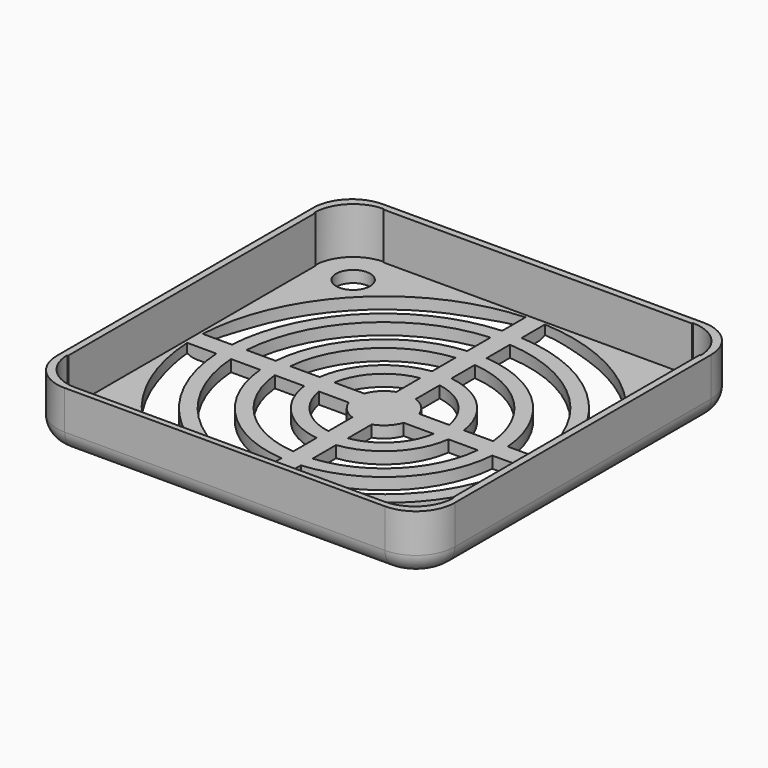
from build123d import *

# Parameters (mm, degrees)
F0_R         = 1.75
F1_DEPTH     = 1.2
F2_DEPTH     = 6
F4_DEPTH     = 10
F5_T1_DEPTH  = 33
F5_T3_DEPTH  = 33
F5_T6_ANGLE  = 90
F5_T8_ANGLE  = 90
F5_T10_ANGLE = 90
F5_T12_ANGLE = 90
F6_DEPTH     = 0.1
F7_DEPTH     = 0.1
F8_DEPTH     = 0.1


# Not quite as in the source:
# - a fillet or chamfer that OpenCascade refuses, or shapes differently, is made with other operations: its cross-section is extruded or revolved along the edge and cut away or added


with BuildPart() as f1:
    # F0 (on Top) → F1 (new body)
    with BuildSketch(Plane.XY):
        with BuildLine():
            Line((-15.9, -19.9), (15.9, -19.9))
            ThreePointArc((15.9, -19.9), (18.7284271247, -18.7284271247), (19.9, -15.9))
            Line((19.9, -15.9), (19.9, 15.9))
            ThreePointArc((19.9, 15.9), (18.7284271247, 18.7284271247), (15.9, 19.9))
            Line((15.9, 19.9), (-15.9, 19.9))
            ThreePointArc((-15.9, 19.9), (-18.7284271247, 18.7284271247), (-19.9, 15.9))
            Line((-19.9, 15.9), (-19.9, -15.9))
            ThreePointArc((-19.9, -15.9), (-18.7284271247, -18.7284271247), (-15.9, -19.9))
        make_face()
        with Locations((-15.9, -15.9)):
            Circle(F0_R, mode=Mode.SUBTRACT)
        with Locations((15.9, -15.9)):
            Circle(F0_R, mode=Mode.SUBTRACT)
        with Locations((-15.9, 15.9)):
            Circle(F0_R, mode=Mode.SUBTRACT)
        with Locations((15.9, 15.9)):
            Circle(F0_R, mode=Mode.SUBTRACT)
    extrude(amount=F1_DEPTH)

    # F0 (on Top) → F2 (join)
    with BuildSketch(Plane.XY):
        with BuildLine():
            Line((-16.5, -20.5), (16.5, -20.5))
            ThreePointArc((16.5, -20.5), (19.3284271247, -19.3284271247), (20.5, -16.5))
            Line((20.5, -16.5), (20.5, 16.5))
            ThreePointArc((20.5, 16.5), (19.3284271247, 19.3284271247), (16.5, 20.5))
            Line((16.5, 20.5), (-16.5, 20.5))
            ThreePointArc((-16.5, 20.5), (-19.3284271247, 19.3284271247), (-20.5, 16.5))
            Line((-20.5, 16.5), (-20.5, -16.5))
            ThreePointArc((-20.5, -16.5), (-19.3284271247, -19.3284271247), (-16.5, -20.5))
        make_face()
        with BuildLine():
            ThreePointArc((19.9, -15.9), (18.7284271247, -18.7284271247), (15.9, -19.9))
            Line((15.9, -19.9), (-15.9, -19.9))
            ThreePointArc((-15.9, -19.9), (-18.7284271247, -18.7284271247), (-19.9, -15.9))
            Line((-19.9, -15.9), (-19.9, 15.9))
            ThreePointArc((-19.9, 15.9), (-18.7284271247, 18.7284271247), (-15.9, 19.9))
            Line((-15.9, 19.9), (15.9, 19.9))
            ThreePointArc((15.9, 19.9), (18.7284271247, 18.7284271247), (19.9, 15.9))
            Line((19.9, 15.9), (19.9, -15.9))
        make_face(mode=Mode.SUBTRACT)
    extrude(amount=F2_DEPTH)

    # F3 (on face) → F4 (cut)
    with BuildSketch(Plane(origin=(0, 0, 0), x_dir=(1, 0, 0), z_dir=(0, 0, -1))):
        with BuildLine():
            ThreePointArc((1, 2.8284271247), (2.1213203436, 2.1213203436), (2.8284271247, 1))
            Line((2.8284271247, 1), (5.9160797831, 1))
            ThreePointArc((5.9160797831, 1), (4.2426406871, 4.2426406871), (1, 5.9160797831))
            Line((1, 5.9160797831), (1, 2.8284271247))
        make_face()
        with BuildLine():
            Line((5.9160797831, -1), (2.8284271247, -1))
            ThreePointArc((2.8284271247, -1), (2.1213203436, -2.1213203436), (1, -2.8284271247))
            Line((1, -2.8284271247), (1, -5.9160797831))
            ThreePointArc((1, -5.9160797831), (4.2426406871, -4.2426406871), (5.9160797831, -1))
        make_face()
        with BuildLine():
            ThreePointArc((-2.8284271247, 1), (-2.1213203436, 2.1213203436), (-1, 2.8284271247))
            Line((-1, 2.8284271247), (-1, 5.9160797831))
            ThreePointArc((-1, 5.9160797831), (-4.2426406871, 4.2426406871), (-5.9160797831, 1))
            Line((-5.9160797831, 1), (-2.8284271247, 1))
        make_face()
        with BuildLine():
            ThreePointArc((1, 7.4330343737), (5.3033008589, 5.3033008589), (7.4330343737, 1))
            Line((7.4330343737, 1), (10.4522724802, 1))
            ThreePointArc((10.4522724802, 1), (7.4246212025, 7.4246212025), (1, 10.4522724802))
            Line((1, 10.4522724802), (1, 7.4330343737))
        make_face()
        with BuildLine():
            Line((-1, -5.9160797831), (-1, -2.8284271247))
            ThreePointArc((-1, -2.8284271247), (-2.1213203436, -2.1213203436), (-2.8284271247, -1))
            Line((-2.8284271247, -1), (-5.9160797831, -1))
            ThreePointArc((-5.9160797831, -1), (-4.2426406871, -4.2426406871), (-1, -5.9160797831))
        make_face()
        with BuildLine():
            Line((10.4522724802, -1), (7.4330343737, -1))
            ThreePointArc((7.4330343737, -1), (5.3033008589, -5.3033008589), (1, -7.4330343737))
            Line((1, -7.4330343737), (1, -10.4522724802))
            ThreePointArc((1, -10.4522724802), (7.4246212025, -7.4246212025), (10.4522724802, -1))
        make_face()
        with BuildLine():
            ThreePointArc((-7.4330343737, 1), (-5.3033008589, 5.3033008589), (-1, 7.4330343737))
            Line((-1, 7.4330343737), (-1, 10.4522724802))
            ThreePointArc((-1, 10.4522724802), (-7.4246212025, 7.4246212025), (-10.4522724802, 1))
            Line((-10.4522724802, 1), (-7.4330343737, 1))
        make_face()
        with BuildLine():
            ThreePointArc((1, 11.9582607431), (8.4852813742, 8.4852813742), (11.9582607431, 1))
            Line((11.9582607431, 1), (14.9666295471, 1))
            ThreePointArc((14.9666295471, 1), (10.6066017178, 10.6066017178), (1, 14.9666295471))
            Line((1, 14.9666295471), (1, 11.9582607431))
        make_face()
        with BuildLine():
            Line((-1, -10.4522724802), (-1, -7.4330343737))
            ThreePointArc((-1, -7.4330343737), (-5.3033008589, -5.3033008589), (-7.4330343737, -1))
            Line((-7.4330343737, -1), (-10.4522724802, -1))
            ThreePointArc((-10.4522724802, -1), (-7.4246212025, -7.4246212025), (-1, -10.4522724802))
        make_face()
        with BuildLine():
            Line((14.9666295471, -1), (11.9582607431, -1))
            ThreePointArc((11.9582607431, -1), (8.4852813742, -8.4852813742), (1, -11.9582607431))
            Line((1, -11.9582607431), (1, -14.9666295471))
            ThreePointArc((1, -14.9666295471), (10.6066017178, -10.6066017178), (14.9666295471, -1))
        make_face()
        with BuildLine():
            ThreePointArc((-11.9582607431, 1), (-8.4852813742, 8.4852813742), (-1, 11.9582607431))
            Line((-1, 11.9582607431), (-1, 14.9666295471))
            ThreePointArc((-1, 14.9666295471), (-10.6066017178, 10.6066017178), (-14.9666295471, 1))
            Line((-14.9666295471, 1), (-11.9582607431, 1))
        make_face()
        with BuildLine():
            ThreePointArc((1, 16.469669092), (11.6672618896, 11.6672618896), (16.469669092, 1))
            Line((16.469669092, 1), (19.4743420942, 1))
            ThreePointArc((19.4743420942, 1), (13.7885822331, 13.7885822331), (1, 19.4743420942))
            Line((1, 19.4743420942), (1, 16.469669092))
        make_face()
        with BuildLine():
            Line((-1, -14.9666295471), (-1, -11.9582607431))
            ThreePointArc((-1, -11.9582607431), (-8.4852813742, -8.4852813742), (-11.9582607431, -1))
            Line((-11.9582607431, -1), (-14.9666295471, -1))
            ThreePointArc((-14.9666295471, -1), (-10.6066017178, -10.6066017178), (-1, -14.9666295471))
        make_face()
        with BuildLine():
            Line((19.4743420942, -1), (16.469669092, -1))
            ThreePointArc((16.469669092, -1), (11.6672618896, -11.6672618896), (1, -16.469669092))
            Line((1, -16.469669092), (1, -19.4743420942))
            ThreePointArc((1, -19.4743420942), (13.7885822331, -13.7885822331), (19.4743420942, -1))
        make_face()
        with BuildLine():
            ThreePointArc((-16.469669092, 1), (-11.6672618896, 11.6672618896), (-1, 16.469669092))
            Line((-1, 16.469669092), (-1, 19.4743420942))
            ThreePointArc((-1, 19.4743420942), (-13.7885822331, 13.7885822331), (-19.4743420942, 1))
            Line((-19.4743420942, 1), (-16.469669092, 1))
        make_face()
        with BuildLine():
            Line((-1, -19.4743420942), (-1, -16.469669092))
            ThreePointArc((-1, -16.469669092), (-11.6672618896, -11.6672618896), (-16.469669092, -1))
            Line((-16.469669092, -1), (-19.4743420942, -1))
            ThreePointArc((-19.4743420942, -1), (-13.7885822331, -13.7885822331), (-1, -19.4743420942))
        make_face()
    extrude(amount=-F4_DEPTH, mode=Mode.SUBTRACT)

    # F5: fillet of radius 2 on 8 edges, made by hand

    # F5_s2 → F5_t1 (cut)
    with BuildSketch(Plane.YZ.offset(-16.5)):
        with BuildLine():
            ThreePointArc((-18.5, 0), (-19.9142135624, 0.5857864376), (-20.5, 2))
            Line((-20.5, 2), (-20.5, 0))
            Line((-20.5, 0), (-18.5, 0))
        make_face()
        with BuildLine():
            ThreePointArc((18.5, 0), (19.9142135624, 0.5857864376), (20.5, 2))
            Line((20.5, 2), (20.5, 0))
            Line((20.5, 0), (18.5, 0))
        make_face()
    extrude(amount=F5_T1_DEPTH, mode=Mode.SUBTRACT)

    # F5_s4 → F5_t3 (cut)
    with BuildSketch(Plane.XZ.offset(-16.5)):
        with BuildLine():
            ThreePointArc((-18.5, 0), (-19.9142135624, 0.5857864376), (-20.5, 2))
            Line((-20.5, 2), (-20.5, 0))
            Line((-20.5, 0), (-18.5, 0))
        make_face()
        with BuildLine():
            ThreePointArc((18.5, 0), (19.9142135624, 0.5857864376), (20.5, 2))
            Line((20.5, 2), (20.5, 0))
            Line((20.5, 0), (18.5, 0))
        make_face()
    extrude(amount=F5_T3_DEPTH, mode=Mode.SUBTRACT)

    # F5_s5 → F5_t6 (revolve, cut)
    with BuildSketch(Plane.XZ.offset(16.5)):
        with BuildLine():
            ThreePointArc((-18.5, 0), (-19.9142135624, 0.5857864376), (-20.5, 2))
            Line((-20.5, 2), (-20.5, 0))
            Line((-20.5, 0), (-18.5, 0))
        make_face()
    revolve(axis=Axis((-16.5, -16.5, 0), (0, 0, 1)), revolution_arc=F5_T6_ANGLE, mode=Mode.SUBTRACT)

    # F5_s7 → F5_t8 (revolve, cut)
    with BuildSketch(Plane.YZ.offset(16.5)):
        with BuildLine():
            ThreePointArc((-18.5, 0), (-19.9142135624, 0.5857864376), (-20.5, 2))
            Line((-20.5, 2), (-20.5, 0))
            Line((-20.5, 0), (-18.5, 0))
        make_face()
    revolve(axis=Axis((16.5, -16.5, 0), (0, 0, 1)), revolution_arc=F5_T8_ANGLE, mode=Mode.SUBTRACT)

    # F5_s9 → F5_t10 (revolve, cut)
    with BuildSketch(Plane.XZ.offset(-16.5)):
        with BuildLine():
            ThreePointArc((18.5, 0), (19.9142135624, 0.5857864376), (20.5, 2))
            Line((20.5, 2), (20.5, 0))
            Line((20.5, 0), (18.5, 0))
        make_face()
    revolve(axis=Axis((16.5, 16.5, 0), (0, 0, 1)), revolution_arc=F5_T10_ANGLE, mode=Mode.SUBTRACT)

    # F5_s11 → F5_t12 (revolve, cut)
    with BuildSketch(Plane.YZ.offset(-16.5)):
        with BuildLine():
            ThreePointArc((18.5, 0), (19.9142135624, 0.5857864376), (20.5, 2))
            Line((20.5, 2), (20.5, 0))
            Line((20.5, 0), (18.5, 0))
        make_face()
    revolve(axis=Axis((-16.5, 16.5, 0), (0, 0, 1)), revolution_arc=F5_T12_ANGLE, mode=Mode.SUBTRACT)

    # F6 (add): a face of the model
    f6_faces = [f1.faces().sort_by_distance(p)[0] for p in [
        (19.9, 0, 3.6),
    ]]
    extrude(f6_faces, amount=F6_DEPTH)

    # F7 (add): a face of the model
    f7_faces = [f1.faces().sort_by_distance(p)[0] for p in [
        (-19.9, 0, 3.6),
    ]]
    extrude(f7_faces, amount=F7_DEPTH)

    # F8 (add): a face of the model
    f8_faces = [f1.faces().sort_by_distance(p)[0] for p in [
        (0, 19.9, 3.6),
    ]]
    extrude(f8_faces, amount=F8_DEPTH)


solid = f1.part
